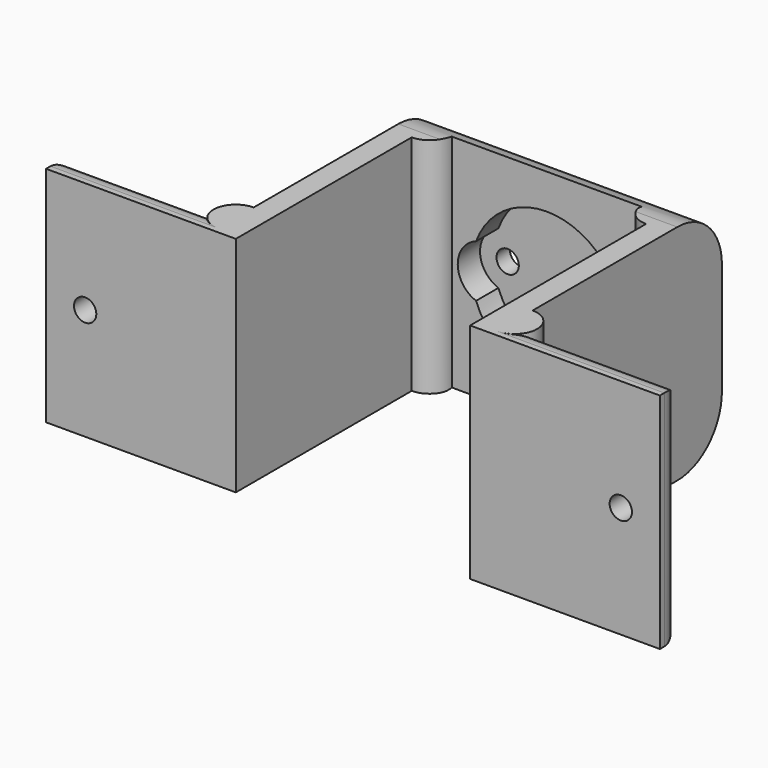
from build123d import *
from build123d import SkipClean  # not in build123d's __all__

# Parameters (mm, degrees)
F0_W         = 25
F0_H         = 20
F1_DEPTH     = 4
F2_R         = 6.75
F3_DEPTH     = 2.5
F5_DEPTH     = 3
F6_R         = 1
F7_DEPTH     = 25
F9_DEPTH     = 2.5
F10_W        = 2
F10_H        = 20
F11_DEPTH    = 21.7
F12_W        = 2.5
F12_H        = 20
F13_DEPTH    = 15
F14_W        = 2.5
F14_H        = 20
F15_DEPTH    = 15
F16_R        = 2
F17_DEPTH    = 20
F18_T1_DEPTH = 50
F19_R        = 2
F20_R        = 1
F21_DEPTH    = 25


# Not quite as in the source:
# - a fillet or chamfer that OpenCascade refuses, or shapes differently, is made with other operations: its cross-section is extruded or revolved along the edge and cut away or added


with BuildPart() as f1:
    # F0 (on Front) → F1 (new body)
    with BuildSketch(Plane.XZ):
        Rectangle(F0_W, F0_H)
    extrude(amount=F1_DEPTH)

    # F2 (on face) → F3 (cut)
    with BuildSketch(Plane.XZ.offset(4)):
        Circle(F2_R)
    extrude(amount=-F3_DEPTH, mode=Mode.SUBTRACT)

    # F4 (on face) → F5 (cut)
    with BuildSketch(Plane.XZ.offset(4)):
        with BuildLine():
            Line((-1.5, -10), (1.5, -10))
            Line((1.5, -10), (1.5, -6.5812232905))
            ThreePointArc((1.5, -6.5812232905), (0, -6.75), (-1.5, -6.5812232905))
            Line((-1.5, -6.5812232905), (-1.5, -10))
        make_face()
    extrude(amount=-F5_DEPTH, mode=Mode.SUBTRACT)

    # F6 (on face) → F7 (cut)
    with BuildSketch(Plane.XZ.offset(1.5)):
        with Locations((-5.5, 0)):
            Circle(F6_R)
        with BuildLine():
            ThreePointArc((6.5, 0), (5.5, 1), (4.5, 0))
            ThreePointArc((4.5, 0), (5.5, -1), (6.5, 0))
        make_face()
    extrude(amount=-F7_DEPTH, mode=Mode.SUBTRACT)

    # F8 (on face) → F9 (cut)
    with BuildSketch(Plane.XZ.offset(4)):
        with BuildLine():
            ThreePointArc((-6.3279938101, -2.3492539963), (-6.75, 0), (-6.3279938101, 2.3492539963))
            ThreePointArc((-6.3279938101, 2.3492539963), (-7.9730051197, 0), (-6.3279938101, -2.3492539963))
        make_face()
        with BuildLine():
            ThreePointArc((6.3071160898, -2.4047425289), (6.75, 0), (6.3071160898, 2.4047425289))
            ThreePointArc((6.3071160898, 2.4047425289), (3.1235860102, 0), (6.3071160898, -2.4047425289))
        make_face()
        with BuildLine():
            ThreePointArc((8.1235860102, 0), (7.6184325204, 1.5068468404), (6.3071160898, 2.4047425289))
            ThreePointArc((6.3071160898, 2.4047425289), (6.75, 0), (6.3071160898, -2.4047425289))
            ThreePointArc((6.3071160898, -2.4047425289), (7.6184325204, -1.5068468404), (8.1235860102, 0))
        make_face()
    extrude(amount=-F9_DEPTH, mode=Mode.SUBTRACT)

    # F10 (on face) → F11 (join)
    with BuildSketch(Plane.XZ.offset(4)):
        with Locations((-11.5, 0)):
            Rectangle(F10_W, F10_H)
        with Locations((11.5, 0)):
            Rectangle(F10_W, F10_H)
    extrude(amount=F11_DEPTH)

    # F12 (on face) → F13 (join)
    with BuildSketch(Plane.YZ.offset(12.5)):
        with Locations((-24.45, 0)):
            Rectangle(F12_W, F12_H)
    extrude(amount=F13_DEPTH)

    # F14 (on face) → F15 (join)
    with BuildSketch(Plane(origin=(-12.5, 0, 0), x_dir=(0, -1, 0), z_dir=(-1, 0, 0))):
        with Locations((24.45, 0)):
            Rectangle(F14_W, F14_H)
    extrude(amount=F15_DEPTH)

    # F16 (on face) → F17 (join)
    with BuildSketch(Plane(origin=(0, 0, -10), x_dir=(1, 0, 0), z_dir=(0, 0, -1))):
        with Locations((-12.5, 23.2)):
            Circle(F16_R)
        with Locations((12.5, 23.2)):
            Circle(F16_R)
        with Locations((-10.5, 4)):
            Circle(F16_R)
        with Locations((10.5, 4)):
            Circle(F16_R)
    extrude(amount=-F17_DEPTH)

    # F18: fillet of radius 5 on 2 edges, made by hand

    # F18_s2 → F18_t1 (cut)
    with BuildSketch(Plane.YZ.offset(-25)):
        with BuildLine():
            ThreePointArc((-5, 10), (-1.4644660941, 8.5355339059), (0, 5))
            Line((0, 5), (0, 10))
            Line((0, 10), (-5, 10))
        make_face()
        with BuildLine():
            ThreePointArc((-5, -10), (-1.4644660941, -8.5355339059), (0, -5))
            Line((0, -5), (0, -10))
            Line((0, -10), (-5, -10))
        make_face()
    extrude(amount=F18_T1_DEPTH, mode=Mode.SUBTRACT)

    # F19
    f19_edges = [f1.edges().sort_by_distance(p)[0] for p in [
        (21, -23.2, -10),
        (21, -23.2, 10),
        (-21, -23.2, -10),
        (-21, -23.2, 10),
        (27.5, -23.2, 0),
        (-27.5, -23.2, 0),
    ]]
    fillet(f19_edges, radius=F19_R)

    # F20 (on face) → F21 (cut)
    with BuildSketch(Plane.XZ.offset(25.7)):
        with Locations((-24, 0)):
            Circle(F20_R)
        with BuildLine():
            ThreePointArc((25, 0), (24, 1), (23, 0))
            ThreePointArc((23, 0), (24, -1), (25, 0))
        make_face()
    with SkipClean():  # cleaning this boolean's faces spoils the solid; the shape is the same uncleaned
        extrude(amount=-F21_DEPTH, mode=Mode.SUBTRACT)


solid = f1.part
